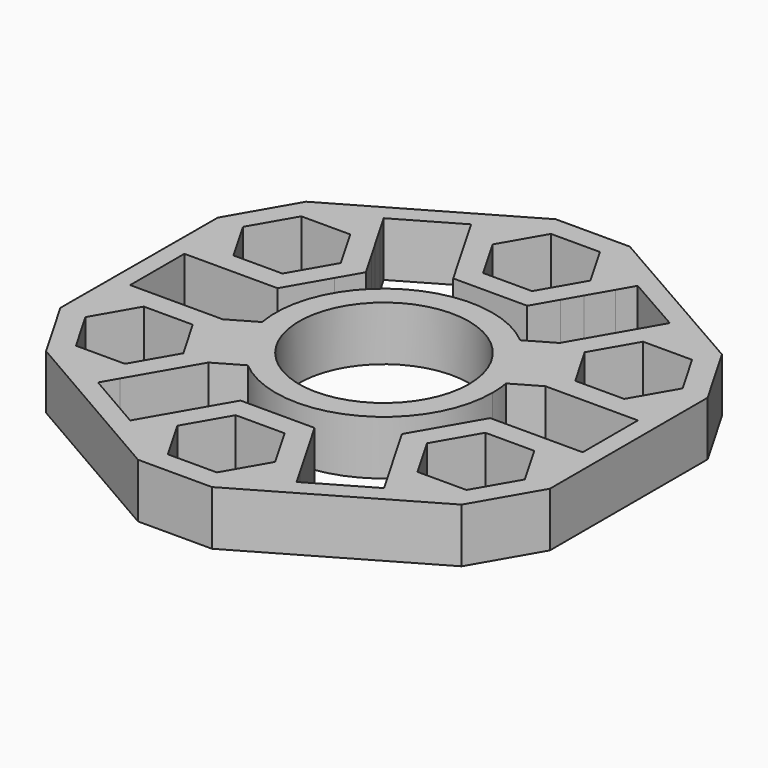
from build123d import *

# Parameters (mm, degrees)
F0_R     = 11.0786603321
F0_R_2   = 10.9474
F1_DEPTH = 6.9977
F2_R     = 13.2854455685
F2_R_2   = 11.176
F3_DEPTH = 6.9977


# Not quite as in the source:
# - a feature names something its author has since deleted; it is built from what else it names


with BuildPart() as f1:
    # F0 (on Top) → F1 (new body)
    with BuildSketch(Plane.XY):
        with BuildLine():
            ThreePointArc((8.9895158912, 10.693432753), (-6.985, 12.0983748909), (-13.7555423633, -2.438432753))
            ThreePointArc((-13.7555423633, -2.438432753), (-12.0983748909, -6.985), (-8.9895158912, -10.693432753))
            ThreePointArc((-8.9895158912, -10.693432753), (5.8981930708, -12.6638153216), (13.97, 0))
            ThreePointArc((13.97, 0), (13.9162823127, 1.2239226251), (13.7555423633, 2.438432753))
            ThreePointArc((13.7555423633, 2.438432753), (13.347336888, 4.1242572662), (12.7333664349, 5.7465014779))
            ThreePointArc((12.7333664349, 5.7465014779), (11.139521372, 8.4304189458), (8.9895158912, 10.693432753))
        make_face()
        Circle(F0_R, mode=Mode.SUBTRACT)
        Circle(F0_R)
        Circle(F0_R_2, mode=Mode.SUBTRACT)
        Polygon((-14.0807527651, 9.595996083), (-12.3768237899, 12.5472876405), (-14.2130055479, 15.7276477372), (-15.394837026, 17.7746399033), (-17.1428502621, 20.8022876405), (-21.9088767342, 20.8022876405), (-26.6749032064, 20.8022876405), (-31.4409296786, 12.5472876405), (-29.1460849644, 8.5725), (-26.6749032064, 4.2922876405), (-17.1428502621, 4.2922876405), (-15.3507527651, 7.3962915574), align=None)
        Polygon((-18.7559669142, 18.0082876405), (-15.6030570942, 12.5472876405), (-18.7559669142, 7.0862876405), (-25.0617865543, 7.0862876405), (-28.2146963743, 12.5472876405), (-25.0617865543, 18.0082876405), align=None, mode=Mode.SUBTRACT)
        Polygon((4.854194994, 33.5022876405), (-4.6778579503, 33.5022876405), (-7.0608711864, 29.3747876405), (-9.4438844224, 25.2472876405), (-4.6778579503, 16.9922876405), (-1.27, 16.9922876405), (1.27, 16.9922876405), (4.854194994, 16.9922876405), (6.6462924911, 20.0962915574), (7.9162924911, 22.295996083), (9.6202214662, 25.2472876405), (7.2372082301, 29.3747876405), align=None)
        Polygon((6.393988162, 25.2472876405), (3.2410783419, 19.7862876405), (-3.0647412982, 19.7862876405), (-6.2176511182, 25.2472876405), (-3.0647412982, 30.7082876405), (3.2410783419, 30.7082876405), align=None, mode=Mode.SUBTRACT)
        Polygon((-29.1460849644, -8.5725), (-31.5290982004, -12.7), (-26.7630717283, -20.955), (-21.9970452561, -20.955), (-17.231018784, -20.955), (-12.4649923118, -12.7), (-14.2130055479, -9.6723522628), (-15.4830055479, -7.4726477372), (-17.231018784, -4.445), (-20.7270452561, -4.445), (-23.2670452561, -4.445), (-26.7630717283, -4.445), align=None)
        Polygon((-25.150604473, -7.2393749809), (-18.8447848775, -7.2386250963), (-15.6912256606, -12.6992501153), (-18.8434860392, -18.1606250191), (-25.1493056347, -18.1613749037), (-28.3028648516, -12.7007498847), align=None, mode=Mode.SUBTRACT)
        Polygon((31.5290982004, 12.7), (26.7630717283, 20.955), (21.9970452561, 20.955), (17.231018784, 20.955), (12.4649923118, 12.7), (14.2130055479, 9.6723522628), (15.4830055479, 7.4726477372), (17.231018784, 4.445), (20.7270452561, 4.445), (23.2670452561, 4.445), (26.7630717283, 4.445), (29.1460849644, 8.5725), align=None)
        Polygon((25.1499550762, 7.239), (18.8441354361, 7.239), (15.691225616, 12.7), (18.8441354361, 18.161), (25.1499550762, 18.161), (28.3028648962, 12.7), align=None, mode=Mode.SUBTRACT)
        Polygon((-7.1490397082, -29.5275), (-4.7660264722, -33.655), (4.7660264722, -33.655), (7.1490397082, -29.5275), (9.5320529443, -25.4), (4.7660264722, -17.145), (1.27, -17.145), (-1.27, -17.145), (-4.7660264722, -17.145), (-6.5140397082, -20.1726477372), (-7.7840397082, -22.3723522628), (-9.5320529443, -25.4), align=None)
        Polygon((-6.3058196401, -25.4), (-3.15290982, -19.939), (3.15290982, -19.939), (6.3058196401, -25.4), (3.15290982, -30.861), (-3.15290982, -30.861), align=None, mode=Mode.SUBTRACT)
        Polygon((26.7630717283, -20.955), (31.5290982004, -12.7), (29.1460849644, -8.5725), (26.7630717283, -4.445), (17.231018784, -4.445), (12.4649923118, -12.7), (14.2130055479, -15.7276477372), (15.4830055479, -17.9273522628), (17.231018784, -20.955), (21.9970452561, -20.955), align=None)
        Polygon((18.8441354361, -18.161), (15.691225616, -12.7), (18.8441354361, -7.239), (25.1499550762, -7.239), (28.3028648962, -12.7), (25.1499550762, -18.161), align=None, mode=Mode.SUBTRACT)
        Polygon((-26.6749032064, 20.8022876405), (-21.9088767342, 20.8022876405), (-18.3343568801, 22.8660376405), (-10.6353910405, 27.3110376405), (-7.0608711864, 29.3747876405), (-4.6778579503, 33.5022876405), align=None)
        Polygon((-21.9970452561, -20.955), (-26.7630717283, -20.955), (-4.7660264722, -33.655), (-7.1490397082, -29.5275), (-10.7235595624, -27.46375), (-18.422525402, -23.01875), align=None)
        Polygon((31.5290982004, -12.7), (31.5290982004, 12.7), (29.1460849644, 8.5725), (29.1460849644, 4.445), (29.1460849644, -4.445), (29.1460849644, -8.5725), align=None)
        Polygon((7.1490397082, -29.5275), (4.7660264722, -33.655), (26.7630717283, -20.955), (21.9970452561, -20.955), (18.422525402, -23.01875), (10.7235595624, -27.46375), align=None)
        Polygon((26.7630717283, 20.955), (4.854194994, 33.5022876405), (7.2372082301, 29.3747876405), (10.811599772, 27.3357666355), (18.4011736203, 23.0062743808), (21.9970452561, 20.955), align=None)
        Polygon((-29.1460849644, 4.2922876405), (-29.1460849644, 8.5725), (-31.4409296786, 12.5472876405), (-31.5290982004, -12.7), (-29.1460849644, -8.5725), (-29.1460849644, -4.445), align=None)
        with BuildLine():
            Line((-13.7555423633, -2.438432753), (-17.231018784, -4.445))
            Line((-17.231018784, -4.445), (-15.4830055479, -7.4726477372))
            Line((-15.4830055479, -7.4726477372), (-14.2130055479, -9.6723522628))
            Line((-14.2130055479, -9.6723522628), (-12.4649923118, -12.7))
            Line((-12.4649923118, -12.7), (-8.9895158912, -10.693432753))
            ThreePointArc((-8.9895158912, -10.693432753), (-12.0983748909, -6.985), (-13.7555423633, -2.438432753))
        make_face()
        with BuildLine():
            Line((14.2130055479, 9.6723522628), (12.4649923118, 12.7))
            Line((12.4649923118, 12.7), (8.9895158912, 10.693432753))
            ThreePointArc((8.9895158912, 10.693432753), (11.139521372, 8.4304189458), (12.7333664349, 5.7465014779))
            ThreePointArc((12.7333664349, 5.7465014779), (13.347336888, 4.1242572662), (13.7555423633, 2.438432753))
            Line((13.7555423633, 2.438432753), (17.231018784, 4.445))
            Line((17.231018784, 4.445), (15.4830055479, 7.4726477372))
            Line((15.4830055479, 7.4726477372), (14.2130055479, 9.6723522628))
        make_face()
        Polygon((-29.1460849644, 4.2922876405), (-26.6749032064, 4.2922876405), (-29.1460849644, 8.5725), align=None)
        Polygon((10.811599772, 27.3357666355), (7.2372082301, 29.3747876405), (9.6202214662, 25.2472876405), align=None)
        Polygon((-21.9088767342, 20.8022876405), (-17.1428502621, 20.8022876405), (-18.3343568801, 22.8660376405), align=None)
        Polygon((-7.0608711864, 29.3747876405), (-10.6353910405, 27.3110376405), (-9.4438844224, 25.2472876405), align=None)
        Polygon((29.1460849644, 4.445), (29.1460849644, 8.5725), (26.7630717283, 4.445), align=None)
        Polygon((26.7630717283, -4.445), (29.1460849644, -8.5725), (29.1460849644, -4.445), align=None)
        Polygon((18.422525402, -23.01875), (21.9970452561, -20.955), (17.231018784, -20.955), align=None)
        Polygon((9.5320529443, -25.4), (7.1490397082, -29.5275), (10.7235595624, -27.46375), align=None)
        Polygon((-10.7235595624, -27.46375), (-7.1490397082, -29.5275), (-9.5320529443, -25.4), align=None)
        Polygon((-17.231018784, -20.955), (-21.9970452561, -20.955), (-18.422525402, -23.01875), align=None)
        Polygon((-26.7630717283, -4.445), (-29.1460849644, -4.445), (-29.1460849644, -8.5725), align=None)
        Polygon((17.231018784, 20.955), (21.9970452561, 20.955), (18.4011736203, 23.0062743808), align=None)
    extrude(amount=F1_DEPTH)

    # F2 (on Top) → F3 (join)
    with BuildSketch(Plane.XY):
        Circle(F2_R)
        Circle(F2_R_2, mode=Mode.SUBTRACT)
    extrude(amount=F3_DEPTH)


solid = f1.part
